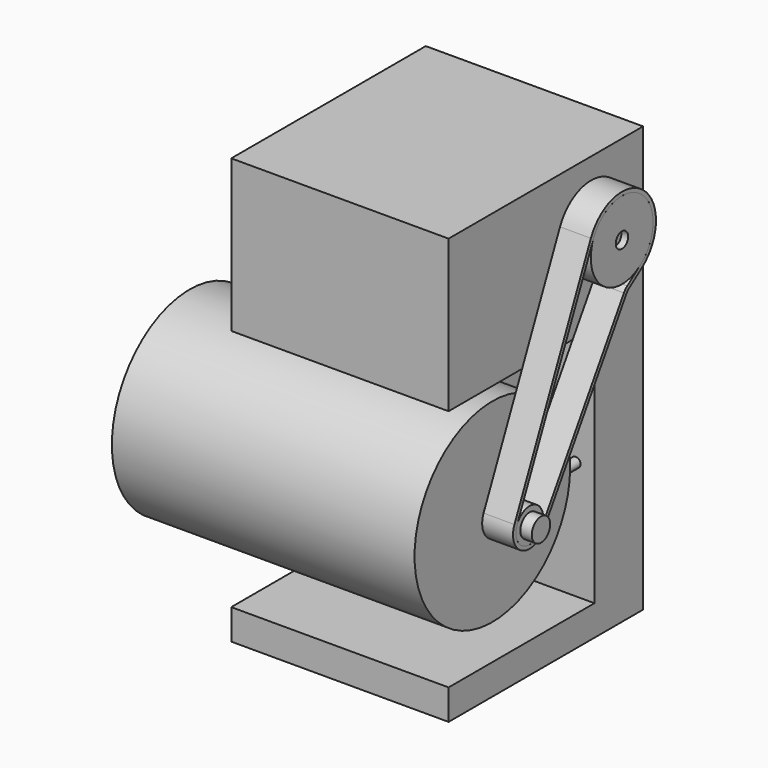
from build123d import *

# Parameters (mm, degrees)
F0_R      = 6.375
F1_DEPTH  = 25
F3_DEPTH  = 178.8
F4_R      = 4
F5_DEPTH  = 22
F6_W      = 7
F6_H      = 22.6
F7_DEPTH  = 3
F8_R      = 80
F9_DEPTH  = 249
F12_DEPTH = 125
F14_R     = 32
F14_R_2   = 6.375
F15_DEPTH = 25.4
F16_R     = 14
F16_R_2   = 9.5
F17_DEPTH = 25.4
F18_R     = 5
F19_DEPTH = 25
F20_R     = 9.5
F21_DEPTH = 40
F23_DEPTH = 25.4


with BuildPart() as f1:
    # F0 (on Right) → F1 (new body)
    with BuildSketch(Plane.YZ):
        with Locations((-10, 126)):
            Circle(F0_R)
    extrude(amount=F1_DEPTH)

    # F2 (on Right) → F3 (join)
    with BuildSketch(Plane.YZ):
        Polygon((0, 49), (0, -151), (-150, -151), (-150, -176), (50, -176), (50, 174), (-150, 174), (-150, 49), align=None)
    extrude(amount=-F3_DEPTH)

    # F4 (on Front) → F5 (join)
    with BuildSketch(Plane.XZ):
        with Locations((-15.4, 0)):
            Circle(F4_R)
        with Locations((-163.4, 0)):
            Circle(F4_R)
        with Locations((-163.4, -54)):
            Circle(F4_R)
        with Locations((-15.4, -54)):
            Circle(F4_R)
    extrude(amount=F5_DEPTH)

    # F6 (on face) → F7 (join)
    with BuildSketch(Plane.XZ):
        with Locations((-3.5, 37.7)):
            Rectangle(F6_W, F6_H)
        with Locations((-175.3, 37.7)):
            Rectangle(F6_W, F6_H)
    extrude(amount=F7_DEPTH)


with BuildPart() as f9:
    # F8 (on Right) → F9 (new body)
    with BuildSketch(Plane.YZ):
        with Locations((-105, -42)):
            Circle(F8_R)
    extrude(amount=-F9_DEPTH)

    # F11 (on offset) → F12 (join)
    with BuildSketch(Plane.YZ.offset(-37.5)):
        with BuildLine():
            Line((-25, 1.5), (-25, 36.5))
            Line((-25, 36.5), (-34, 36.5))
            Line((-34, 36.5), (-53.4142365036, 19.146618913))
            ThreePointArc((-53.4142365036, 19.146618913), (-44.9850899063, 10.8981149612), (-37.8602204353, 1.5))
            Line((-37.8602204353, 1.5), (-25, 1.5))
        make_face()
        with BuildLine():
            Line((-25, -120.5), (-25, -85.5))
            Line((-25, -85.5), (-37.8602204353, -85.5))
            ThreePointArc((-37.8602204353, -85.5), (-44.9850899063, -94.8981149612), (-53.4142365036, -103.146618913))
            Line((-53.4142365036, -103.146618913), (-34, -120.5))
            Line((-34, -120.5), (-25, -120.5))
        make_face()
    extrude(amount=-F12_DEPTH)

    # F18 (on face) → F19 (cut)
    with BuildSketch(Plane(origin=(0, -25, 0), x_dir=(-1, 0, 0), z_dir=(0, 1, 0))):
        with Locations((50, 20.5)):
            Circle(F18_R)
        with Locations((150, 20.5)):
            Circle(F18_R)
        with Locations((150, -104.5)):
            Circle(F18_R)
        with Locations((50, -104.5)):
            Circle(F18_R)
    extrude(amount=-F19_DEPTH, mode=Mode.SUBTRACT)

    # F20 (on face) → F21 (join)
    with BuildSketch(Plane.YZ):
        with Locations((-105, -42)):
            Circle(F20_R)
    extrude(amount=F21_DEPTH)


with BuildPart() as f15:
    # F14 (on offset) → F15 (new body)
    with BuildSketch(Plane.YZ.offset(30.6)):
        with Locations((-10, 126)):
            Circle(F14_R)
        with Locations((-10, 126)):
            Circle(F14_R_2, mode=Mode.SUBTRACT)
    extrude(amount=-F15_DEPTH)


with BuildPart() as f17:
    # F16 (on offset) → F17 (new body)
    with BuildSketch(Plane.YZ.offset(30.6)):
        with Locations((-105, -42)):
            Circle(F16_R)
        with Locations((-105, -42)):
            Circle(F16_R_2, mode=Mode.SUBTRACT)
    extrude(amount=-F17_DEPTH)


with BuildPart() as f23:
    # F22 (on offset) → F23 (new body)
    with BuildSketch(Plane.YZ.offset(30.6)):
        with BuildLine():
            Line((-41.940285012, 140.3114706913), (-120.5138527201, -35.0487142356))
            ThreePointArc((-120.5138527201, -35.0487142356), (-112.9985919726, -57.000750863), (-90.5829491892, -51.0082543215))
            Line((-90.5829491892, -51.0082543215), (-5.4136460596, 85.2989731303))
            ThreePointArc((-5.4136460596, 85.2989731303), (-4.2247545268, 86.8432976933), (-2.7588939467, 88.1276863388))
            Line((-2.7588939467, 88.1276863388), (10.3905310387, 97.5530978144))
            ThreePointArc((10.3905310387, 97.5530978144), (12.1454017119, 153.1031581742), (-41.940285012, 140.3114706913))
        make_face()
        with BuildLine():
            ThreePointArc((-39.2025462967, 139.0847732035), (10.2472244223, 150.7800303307), (8.6427712354, 99.991403716))
            Line((8.6427712354, 99.991403716), (-4.50665375, 90.5659922404))
            ThreePointArc((-4.50665375, 90.5659922404), (-6.4122725042, 88.8962870013), (-7.9578314968, 86.8886650693))
            Line((-7.9578314968, 86.8886650693), (-93.1271346264, -49.4185623824))
            ThreePointArc((-93.1271346264, -49.4185623824), (-111.5870757422, -54.3535595343), (-117.7761140048, -36.2754117235))
            Line((-117.7761140048, -36.2754117235), (-39.2025462967, 139.0847732035))
        make_face(mode=Mode.SUBTRACT)
    extrude(amount=-F23_DEPTH)


solid = Compound([f1.part, f9.part, f15.part, f17.part, f23.part])
